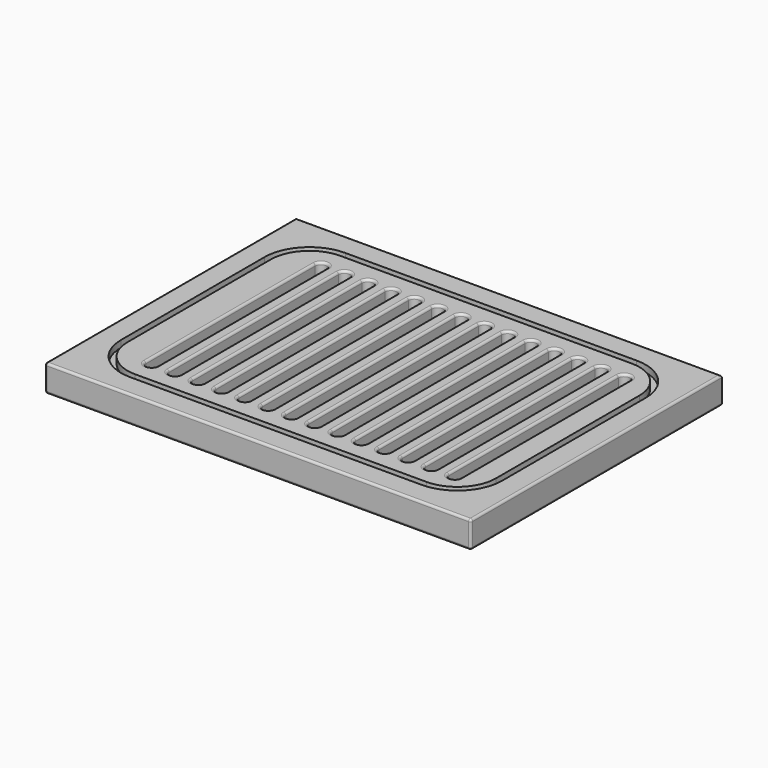
from build123d import *

# Parameters (mm, degrees)
F0_W     = 241.3
F0_H     = 177.8
F2_DEPTH = 15.24
F5_DEPTH = 3.81
F7_DEPTH = 3.81
F9_DEPTH = 15.241
F11_R    = 1.27
F12_R    = 1.27


# Not quite as in the source:
# - a variable given as a bare number and used for a length is read in inches; the dataset says mm whatever the document's units were
# - ends of sketch curves that miss each other by under 0.0002 mm in the source are joined


with BuildPart() as f2:
    # F0 (on Top) → F2 (new body)
    with BuildSketch(Plane.XY):
        with Locations((120.65, 88.9)):
            Rectangle(F0_W, F0_H)
    extrude(amount=F2_DEPTH)

    # F3 (on face) → F5 (cut)
    with BuildSketch(Plane.XY.offset(15.24)):
        with BuildLine():
            ThreePointArc((228.6, 139.7), (221.1605122421, 157.6605122421), (203.2, 165.1))
            Line((203.2, 165.1), (38.1, 165.1))
            ThreePointArc((38.1, 165.1), (20.1394884556, 157.6605129398), (12.7, 139.7000019734))
            Line((12.7, 139.7000019734), (12.7, 38.0999988256))
            ThreePointArc((12.7, 38.0999988256), (20.1394881731, 20.1394873427), (38.1, 12.7))
            Line((38.1, 12.7), (203.2, 12.7))
            ThreePointArc((203.2, 12.7), (221.1604988957, 20.1394744114), (228.6, 38.0999622505))
            Line((228.6, 38.0999622505), (228.6, 139.7))
        make_face()
        with BuildLine():
            Line((16.256, 38.0999988256), (16.256, 139.7000019734))
            ThreePointArc((16.256, 139.7000019734), (22.6539601695, 155.1460412259), (38.1, 161.544))
            Line((38.1, 161.544), (203.2, 161.544))
            ThreePointArc((203.2, 161.544), (218.6460395603, 155.1460414962), (225.044, 139.7000027378))
            Line((225.044, 139.7000027378), (225.044, 38.0999649883))
            ThreePointArc((225.044, 38.0999649883), (218.6460281497, 22.6539470932), (203.2, 16.256))
            Line((203.2, 16.256), (38.1, 16.256))
            ThreePointArc((38.1, 16.256), (22.653959887, 22.6539590566), (16.256, 38.0999988256))
        make_face(mode=Mode.SUBTRACT)
    extrude(amount=-F5_DEPTH, mode=Mode.SUBTRACT)

    # F6 (on face) → F7 (cut)
    with BuildSketch(Plane(origin=(0, 0, 0), x_dir=(1, 0, 0), z_dir=(0, 0, -1))):
        with BuildLine():
            ThreePointArc((228.6, -38.099991886), (221.1605122421, -20.1394796439), (203.2, -12.699991886))
            Line((203.2, -12.699991886), (38.1, -12.7000000982))
            ThreePointArc((38.1, -12.7000000982), (20.1394877579, -20.1394834799), (12.7, -38.099995722))
            Line((12.7, -38.099995722), (12.7, -139.7))
            ThreePointArc((12.7, -139.7), (20.1394877579, -157.6605122421), (38.1, -165.1))
            Line((38.1, -165.1), (203.2, -165.1))
            ThreePointArc((203.2, -165.1), (221.1605122421, -157.6605122421), (228.6, -139.7))
            Line((228.6, -139.7), (228.6, -38.099991886))
        make_face()
        with BuildLine():
            Line((16.256, -139.7), (16.256, -38.099995722))
            ThreePointArc((16.256, -38.099995722), (22.6539594718, -22.6539551938), (38.1, -16.255995722))
            Line((38.1, -16.255995722), (203.2, -16.2560000982))
            ThreePointArc((203.2, -16.2560000982), (218.6460405282, -22.6539513578), (225.044, -38.099991886))
            Line((225.044, -38.099991886), (225.044, -139.7))
            ThreePointArc((225.044, -139.7), (218.6460405282, -155.1460405282), (203.2, -161.544))
            Line((203.2, -161.544), (38.1, -161.544))
            ThreePointArc((38.1, -161.544), (22.6539594718, -155.1460405282), (16.256, -139.7))
        make_face(mode=Mode.SUBTRACT)
    extrude(amount=-F7_DEPTH, mode=Mode.SUBTRACT)

    # F8 (on face) → F9 (cut, through all)
    with BuildSketch(Plane(origin=(0, 0, 0), x_dir=(1, 0, 0), z_dir=(0, 0, -1))):
        with BuildLine():
            Line((205.74, -28.956), (205.74, -148.844))
            ThreePointArc((205.74, -148.844), (209.042, -152.146), (212.344, -148.844))
            Line((212.344, -148.844), (212.344, -28.956))
            ThreePointArc((212.344, -28.956), (209.042, -25.654), (205.74, -28.956))
        make_face()
        with BuildLine():
            Line((199.136, -148.844), (199.136, -28.956))
            ThreePointArc((199.136, -28.956), (195.834, -25.654), (192.532, -28.956))
            Line((192.532, -28.956), (192.532, -148.844))
            ThreePointArc((192.532, -148.844), (195.834, -152.146), (199.136, -148.844))
        make_face()
        with BuildLine():
            Line((185.928, -148.844), (185.928, -28.956))
            ThreePointArc((185.928, -28.956), (182.626, -25.654), (179.324, -28.956))
            Line((179.324, -28.956), (179.324, -148.844))
            ThreePointArc((179.324, -148.844), (182.626, -152.146), (185.928, -148.844))
        make_face()
        with BuildLine():
            Line((172.72, -148.844), (172.72, -28.956))
            ThreePointArc((172.72, -28.956), (169.418, -25.654), (166.116, -28.956))
            Line((166.116, -28.956), (166.116, -148.844))
            ThreePointArc((166.116, -148.844), (169.418, -152.146), (172.72, -148.844))
        make_face()
        with BuildLine():
            Line((159.512, -148.844), (159.512, -28.956))
            ThreePointArc((159.512, -28.956), (156.21, -25.654), (152.908, -28.956))
            Line((152.908, -28.956), (152.908, -148.844))
            ThreePointArc((152.908, -148.844), (156.21, -152.146), (159.512, -148.844))
        make_face()
        with BuildLine():
            Line((146.304, -148.844), (146.304, -28.956))
            ThreePointArc((146.304, -28.956), (143.002, -25.654), (139.7, -28.956))
            Line((139.7, -28.956), (139.7, -148.844))
            ThreePointArc((139.7, -148.844), (143.002, -152.146), (146.304, -148.844))
        make_face()
        with BuildLine():
            Line((133.096, -148.844), (133.096, -28.956))
            ThreePointArc((133.096, -28.956), (129.794, -25.654), (126.492, -28.956))
            Line((126.492, -28.956), (126.492, -148.844))
            ThreePointArc((126.492, -148.844), (129.794, -152.146), (133.096, -148.844))
        make_face()
        with BuildLine():
            Line((119.888, -148.844), (119.888, -28.956))
            ThreePointArc((119.888, -28.956), (116.586, -25.654), (113.284, -28.956))
            Line((113.284, -28.956), (113.284, -148.844))
            ThreePointArc((113.284, -148.844), (116.586, -152.146), (119.888, -148.844))
        make_face()
        with BuildLine():
            Line((106.68, -148.844), (106.68, -28.956))
            ThreePointArc((106.68, -28.956), (103.378, -25.654), (100.076, -28.956))
            Line((100.076, -28.956), (100.076, -148.844))
            ThreePointArc((100.076, -148.844), (103.378, -152.146), (106.68, -148.844))
        make_face()
        with BuildLine():
            Line((93.472, -148.844), (93.472, -28.956))
            ThreePointArc((93.472, -28.956), (90.17, -25.654), (86.868, -28.956))
            Line((86.868, -28.956), (86.868, -148.844))
            ThreePointArc((86.868, -148.844), (90.17, -152.146), (93.472, -148.844))
        make_face()
        with BuildLine():
            Line((80.264, -148.844), (80.264, -28.956))
            ThreePointArc((80.264, -28.956), (76.962, -25.654), (73.66, -28.956))
            Line((73.66, -28.956), (73.66, -148.844))
            ThreePointArc((73.66, -148.844), (76.962, -152.146), (80.264, -148.844))
        make_face()
        with BuildLine():
            Line((67.056, -148.844), (67.056, -28.956))
            ThreePointArc((67.056, -28.956), (63.754, -25.654), (60.452, -28.956))
            Line((60.452, -28.956), (60.452, -148.844))
            ThreePointArc((60.452, -148.844), (63.754, -152.146), (67.056, -148.844))
        make_face()
        with BuildLine():
            Line((53.848, -148.844), (53.848, -28.956))
            ThreePointArc((53.848, -28.956), (50.546, -25.654), (47.244, -28.956))
            Line((47.244, -28.956), (47.244, -148.844))
            ThreePointArc((47.244, -148.844), (50.546, -152.146), (53.848, -148.844))
        make_face()
        with BuildLine():
            Line((40.64, -148.844), (40.64, -28.956))
            ThreePointArc((40.64, -28.956), (37.338, -25.654), (34.036, -28.956))
            Line((34.036, -28.956), (34.036, -148.844))
            ThreePointArc((34.036, -148.844), (37.338, -152.146), (40.64, -148.844))
        make_face()
    extrude(amount=-F9_DEPTH, mode=Mode.SUBTRACT)

    # F11
    f11_edges = [f2.edges().sort_by_distance(p)[0] for p in [
        (34.036, 88.9, 15.24),
        (40.64, 88.9, 15.24),
        (47.244, 88.9, 15.24),
        (53.848, 88.9, 15.24),
        (60.452, 88.9, 15.24),
        (67.056, 88.9, 15.24),
        (73.66, 88.9, 15.24),
        (80.264, 88.9, 15.24),
        (86.868, 88.9, 15.24),
        (93.472, 88.9, 15.24),
        (100.076, 88.9, 15.24),
        (106.68, 88.9, 15.24),
        (113.284, 88.9, 15.24),
        (119.888, 88.9, 15.24),
        (126.492, 88.9, 15.24),
        (133.096, 88.9, 15.24),
        (139.7, 88.9, 15.24),
        (146.304, 88.9, 15.24),
        (152.908, 88.9, 15.24),
        (159.512, 88.9, 15.24),
        (166.116, 88.9, 15.24),
        (172.72, 88.9, 15.24),
        (179.324, 88.9, 15.24),
        (185.928, 88.9, 15.24),
        (192.532, 88.9, 15.24),
        (199.136, 88.9, 15.24),
        (205.74, 88.9, 15.24),
        (212.344, 88.9, 15.24),
        (120.65, 0, 0),
        (34.036, 88.9, 0),
        (40.64, 88.9, 0),
        (47.244, 88.9, 0),
        (53.848, 88.9, 0),
        (60.452, 88.9, 0),
        (67.056, 88.9, 0),
        (73.66, 88.9, 0),
        (80.264, 88.9, 0),
        (86.868, 88.9, 0),
        (93.472, 88.9, 0),
        (100.076, 88.9, 0),
        (106.68, 88.9, 0),
        (113.284, 88.9, 0),
        (119.888, 88.9, 0),
        (126.492, 88.9, 0),
        (133.096, 88.9, 0),
        (139.7, 88.9, 0),
        (146.304, 88.9, 0),
        (152.908, 88.9, 0),
        (159.512, 88.9, 0),
        (166.116, 88.9, 0),
        (172.72, 88.9, 0),
        (179.324, 88.9, 0),
        (185.928, 88.9, 0),
        (192.532, 88.9, 0),
        (199.136, 88.9, 0),
        (205.74, 88.9, 0),
        (212.344, 88.9, 0),
    ]]
    fillet(f11_edges, radius=F11_R)

    # F12
    f12_edges = [f2.edges().sort_by_distance(p)[0] for p in [
        (0, 88.9, 15.24),
        (120.65, 177.8, 15.24),
        (241.3, 88.9, 15.24),
        (120.65, 0, 15.24),
        (0, 89.535, 0),
        (120.65, 177.8, 0),
        (120.65, 1.27, 0),
        (241.3, 89.535, 0),
    ]]
    fillet(f12_edges, radius=F12_R)


solid = f2.part
